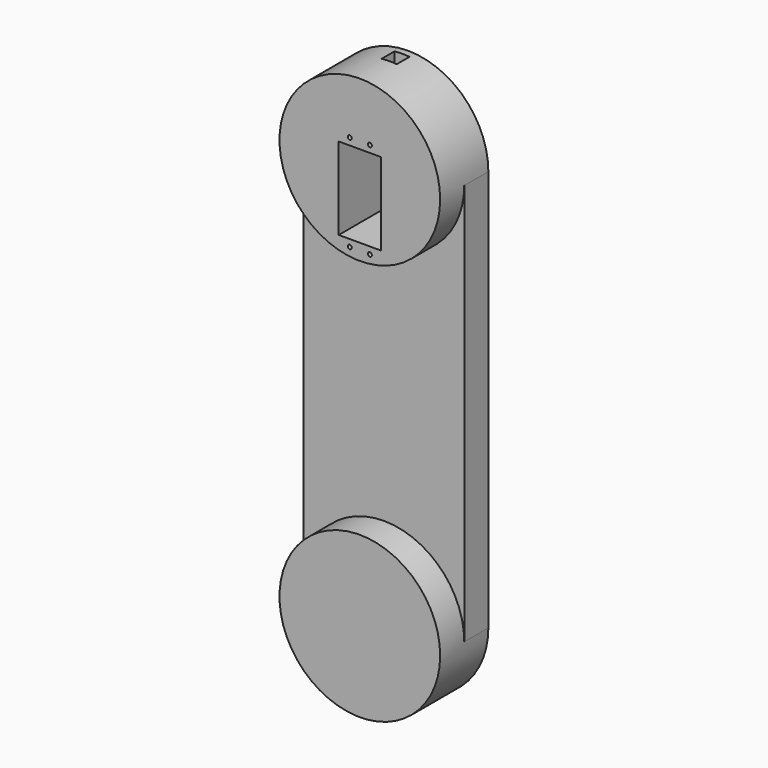
from build123d import *
from build123d import SkipClean  # not in build123d's __all__

# Parameters (mm, degrees)
F1_DEPTH = 15
F2_DEPTH = 15
F3_DEPTH = 15
F4_W     = 21
F4_H     = 41
F5_DEPTH = 26.6
F6_R     = 1
F7_DEPTH = 15
F8_W     = 7.5
F8_H     = 8
F9_DEPTH = 31.001


# Not quite as in the source:
# - after a boolean that leaves OpenCascade's solid faulty, fix() repairs it


with BuildPart() as f1:
    # F0 (on Front) → F1 (new body)
    with BuildSketch(Plane.XZ):
        with BuildLine():
            ThreePointArc((-40, 0), (0, 40), (40, 0))
            Line((40, 0), (40, 200))
            ThreePointArc((40, 200), (0, 160), (-40, 200))
            Line((-40, 200), (-40, 0))
        make_face()
        with BuildLine():
            ThreePointArc((-40, 200), (0, 160), (40, 200))
            ThreePointArc((40, 200), (0, 240), (-40, 200))
        make_face()
        with BuildLine():
            ThreePointArc((-40, 0), (0, -40), (40, 0))
            ThreePointArc((40, 0), (0, 40), (-40, 0))
        make_face()
    extrude(amount=-F1_DEPTH)

    # F0 (on Front) → F2 (join)
    with BuildSketch(Plane.XZ):
        with BuildLine():
            ThreePointArc((-40, 200), (0, 160), (40, 200))
            ThreePointArc((40, 200), (0, 240), (-40, 200))
        make_face()
    with SkipClean():  # cleaning this boolean's faces spoils the solid; the shape is the same uncleaned
        extrude(amount=F2_DEPTH)

    # F0 (on Front) → F3 (join)
    with BuildSketch(Plane.XZ):
        with BuildLine():
            ThreePointArc((-40, 0), (0, -40), (40, 0))
            ThreePointArc((40, 0), (0, 40), (-40, 0))
        make_face()
    with SkipClean():  # cleaning this boolean's faces spoils the solid; the shape is the same uncleaned
        extrude(amount=F3_DEPTH)

    # F4 (on face) → F5 (cut)
    with BuildSketch(Plane.XZ.offset(15)):
        with Locations((0, 188.5)):
            Rectangle(F4_W, F4_H)
    extrude(amount=-F5_DEPTH, mode=Mode.SUBTRACT)

    add(f1.part.fix(), mode=Mode.REPLACE)

    # F6 (on face) → F7 (cut)
    with BuildSketch(Plane.XZ.offset(15)):
        with Locations((-5, 212.5)):
            Circle(F6_R)
        with Locations((5, 212.5)):
            Circle(F6_R)
        with Locations((5, 164.5)):
            Circle(F6_R)
        with Locations((-5, 164.5)):
            Circle(F6_R)
    extrude(amount=-F7_DEPTH, mode=Mode.SUBTRACT)

    # F8 (on face) → F9 (cut, through all)
    with BuildSketch(Plane(origin=(0, 0, 209), x_dir=(1, 0, 0), z_dir=(0, 0, -1))):
        with Locations((-0.25, -7.6)):
            Rectangle(F8_W, F8_H)
    extrude(amount=-F9_DEPTH, mode=Mode.SUBTRACT)


solid = f1.part
